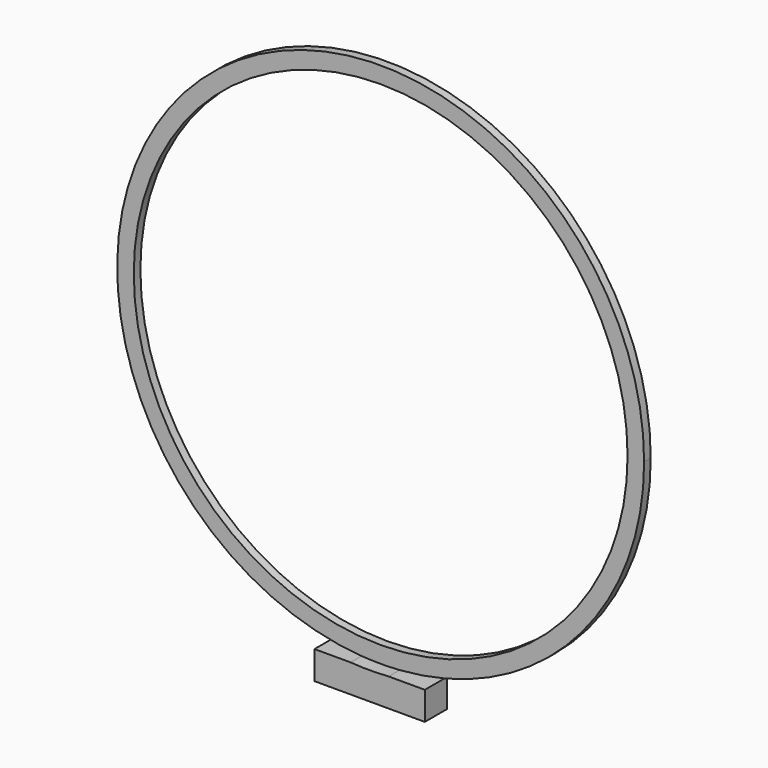
from build123d import *

# Parameters (mm, degrees)
F0_R     = 2425.7
F0_R_2   = 2273.3
F1_DEPTH = 76.2
F3_DEPTH = 127


# Not quite as in the source:
# - a feature of the source that left no trace in its solid (it failed there, or was rolled back) is left out


with BuildPart() as f1:
    # F0 (on Front) → F1 (new body)
    with BuildSketch(Plane.XZ):
        Circle(F0_R)
        Circle(F0_R_2, mode=Mode.SUBTRACT)
    extrude(amount=F1_DEPTH)

    # F2 (on face) → F3 (join, symmetric)
    with BuildSketch(Plane.XZ.offset(76.2)):
        with BuildLine():
            Line((508, -2419.35), (175.402586925, -2419.35))
            ThreePointArc((175.402586925, -2419.35), (0, -2425.7), (-175.402586925, -2419.35))
            Line((-175.402586925, -2419.35), (-508, -2419.35))
            Line((-508, -2419.35), (-508, -2679.7))
            Line((-508, -2679.7), (0, -2679.7))
            Line((0, -2679.7), (508, -2679.7))
            Line((508, -2679.7), (508, -2419.35))
        make_face()
    extrude(amount=F3_DEPTH, both=True)


solid = f1.part
